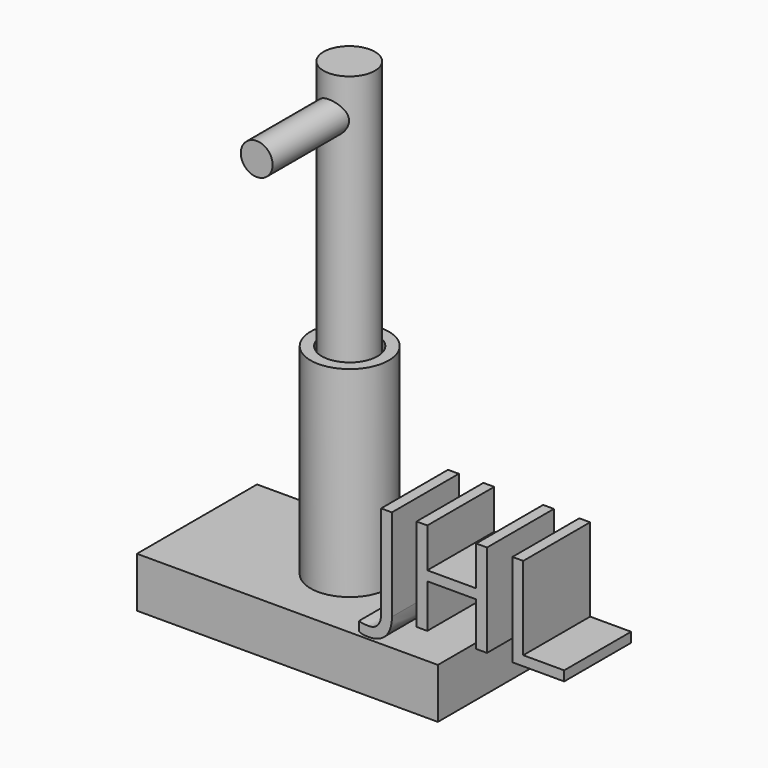
from build123d import *

# Parameters (mm, degrees)
F0_W         = 89.9718813598
F0_H         = 44.8875017464
F0_R         = 11.6825856001
F0_R_2       = 8.3277192609
F1_DEPTH     = 15
F2_DEPTH     = 75
F3_R         = 7.6786357922
F4_DEPTH     = 150
F5_TEXT_SIZE = 38.864199693
F6_DEPTH     = 25
F5_R         = 4.7546853118
F9_DEPTH     = 40


# Not quite as in the source:
# - a feature of the source that left no trace in its solid (it failed there, or was rolled back) is left out
# - Text() gives the source's letters only with a copy of the font that has no kerning and outlines rounded to 1/6400 em; it was checked with that copy


with BuildPart() as f1:
    # F0 (on Top) → F1 (new body)
    with BuildSketch(Plane.XY):
        with Locations((-0.196872279, 34.157814458)):
            Rectangle(F0_W, F0_H)
        with Locations((0, 34.7484387457)):
            Circle(F0_R, mode=Mode.SUBTRACT)
        with Locations((0, 34.7484387457)):
            Circle(F0_R)
        with Locations((0, 34.7484387457)):
            Circle(F0_R_2, mode=Mode.SUBTRACT)
        with Locations((0, 34.7484387457)):
            Circle(F0_R_2)
    extrude(amount=F1_DEPTH)

    # F0 (on Top) → F2 (join)
    with BuildSketch(Plane.XY):
        with Locations((0, 34.7484387457)):
            Circle(F0_R)
        with Locations((0, 34.7484387457)):
            Circle(F0_R_2, mode=Mode.SUBTRACT)
    extrude(amount=F2_DEPTH)


with BuildPart() as f4:
    # F3 (on Top) → F4 (new body)
    with BuildSketch(Plane.XY):
        with Locations((0, 34.583568573)):
            Circle(F3_R)
    extrude(amount=F4_DEPTH)

    # F5 (on Front) → F9 (join)
    with BuildSketch(Plane.XZ):
        with Locations((0, 138.3409500122)):
            Circle(F5_R)
    extrude(amount=-F9_DEPTH)


with BuildPart() as f6:
    # F5 (on Front) → F6 (new body)
    with BuildSketch(Plane.XZ):
        with Locations((53.5830482841, 47.4063716829)):
            Text('JHL', F5_TEXT_SIZE, font='Open Sans', text_align=(TextAlign.LEFT, TextAlign.BOTTOM))
    extrude(amount=F6_DEPTH)


solid = Compound([f1.part, f4.part, f6.part])
